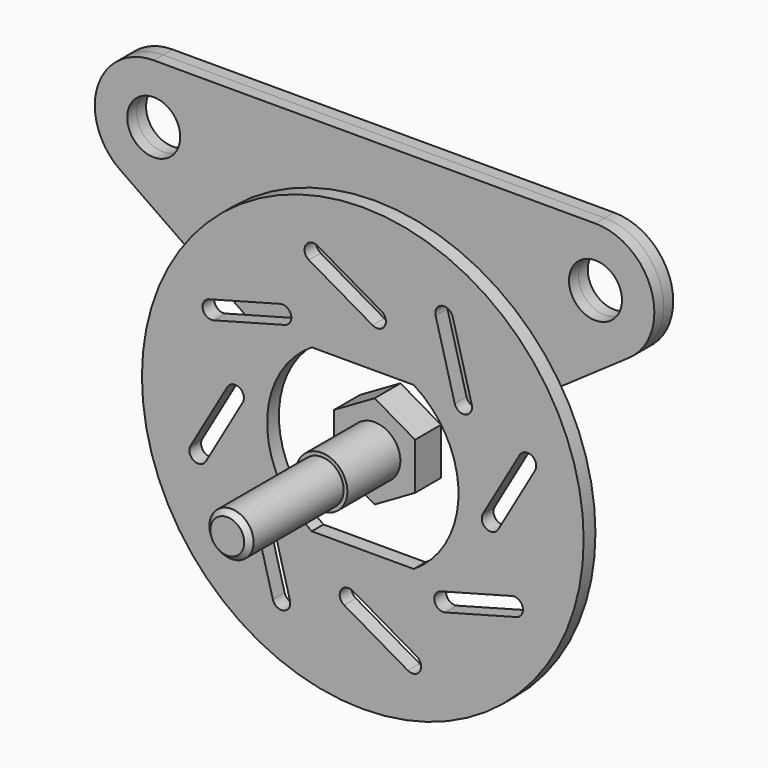
from build123d import *

# Parameters (mm, degrees)
F0_R            = 15
F1_DEPTH        = 1
F3_DEPTH        = 25
F3_COPIES_COUNT = 8
F4_R            = 1.8
F5_DEPTH        = 0.8
F10_DEPTH       = 2.2
F11_SIZE        = 0.35


# Not quite as in the source:
# - a pattern or mirror of a feature is missing from the dataset's text; its kind, count and spacing are read off the source's solid


with BuildPart() as f1:
    # F0 (on Front) → F1 (new body)
    with BuildSketch(Plane.XZ):
        Circle(F0_R)
        with BuildLine():
            ThreePointArc((-3.4641016151, -5.5), (-6.5, 0), (-3.4641016151, 5.5))
            Line((-3.4641016151, 5.5), (3.4641016151, 5.5))
            ThreePointArc((3.4641016151, 5.5), (6.5, 0), (3.4641016151, -5.5))
            Line((3.4641016151, -5.5), (-3.4641016151, -5.5))
        make_face(mode=Mode.SUBTRACT)
    extrude(amount=F1_DEPTH)

    # F2 (on face) → F3 (cut)
    with BuildSketch(Plane.XZ.offset(1)):
        with BuildLine():
            ThreePointArc((-3.0612159322, 11.6978184725), (-3.8808311744, 11.4782032303), (-3.6612159322, 10.658587988))
            Line((-3.6612159322, 10.658587988), (0.6689110868, 8.158587988))
            ThreePointArc((0.6689110868, 8.158587988), (1.488526329, 8.3782032303), (1.2689110868, 9.1978184725))
            Line((1.2689110868, 9.1978184725), (-3.0612159322, 11.6978184725))
        make_face()
    f3 = extrude(amount=-F3_DEPTH, mode=Mode.SUBTRACT)

    # F3_copies: F3 ×8 about axis
    f3_copies_axis = Axis((0, 0, 0), (0, 1, 0))
    for i in range(1, F3_COPIES_COUNT):
        add(f3.rotate(f3_copies_axis, i * 360 / F3_COPIES_COUNT), mode=Mode.SUBTRACT)


with BuildPart() as f5:
    # F4 (on Front) → F5 (new body)
    with BuildSketch(Plane.XZ):
        with BuildLine():
            Line((8.1419410907, 4.8580589093), (17.2838821814, 11.2161178186))
            ThreePointArc((17.2838821814, 11.2161178186), (18.816774078, 15.6967604761), (15, 18.5))
            Line((15, 18.5), (-15, 18.5))
            ThreePointArc((-15, 18.5), (-18.816774078, 15.6967604761), (-17.2838821814, 11.2161178186))
            Line((-17.2838821814, 11.2161178186), (-8.1419410907, 4.8580589093))
            ThreePointArc((-8.1419410907, 4.8580589093), (-6.7856815905, 4.5115162512), (-5.5344130167, 5.1390978013))
            ThreePointArc((-5.5344130167, 5.1390978013), (0, 7.5524865873), (5.5344130167, 5.1390978013))
            ThreePointArc((5.5344130167, 5.1390978013), (6.7856815905, 4.5115162512), (8.1419410907, 4.8580589093))
        make_face()
        with Locations((-15, 14.5)):
            Circle(F4_R, mode=Mode.SUBTRACT)
        with Locations((15, 14.5)):
            Circle(F4_R, mode=Mode.SUBTRACT)
    extrude(amount=-F5_DEPTH)


with BuildPart() as f6_1:
    # F6: copy of F5
    add(f5.part.moved(Location((0, 0.8, 0))))


with BuildPart() as f8:
    # F7 (on Top) → F8 (revolve)
    with BuildSketch(Plane.XY):
        Polygon((0, -12.5), (0, 0), (-1.75, 0), (-1.75, -4.5), (-1.5, -4.5), (-1.5, -12.5), align=None)
    revolve(axis=Axis((0, 0.4439655009, 0), (0, 1, 0)))

    # F9 (on face) → F10 (join)
    with BuildSketch(Plane(origin=(0, 0, 0), x_dir=(-1, 0, 0), z_dir=(0, 1, 0))):
        Polygon((2.75, -1.5877132403), (2.75, 1.5877132403), (0, 3.1754264805), (-2.75, 1.5877132403), (-2.75, -1.5877132403), (0, -3.1754264805), align=None)
    extrude(amount=F10_DEPTH)

    # F11
    f11_edges = [f8.edges().sort_by_distance(p)[0] for p in [
        (1.5, -12.5, 0),
    ]]
    chamfer(f11_edges, length=F11_SIZE)


solid = Compound([f1.part, f5.part, f6_1.part, f8.part])
